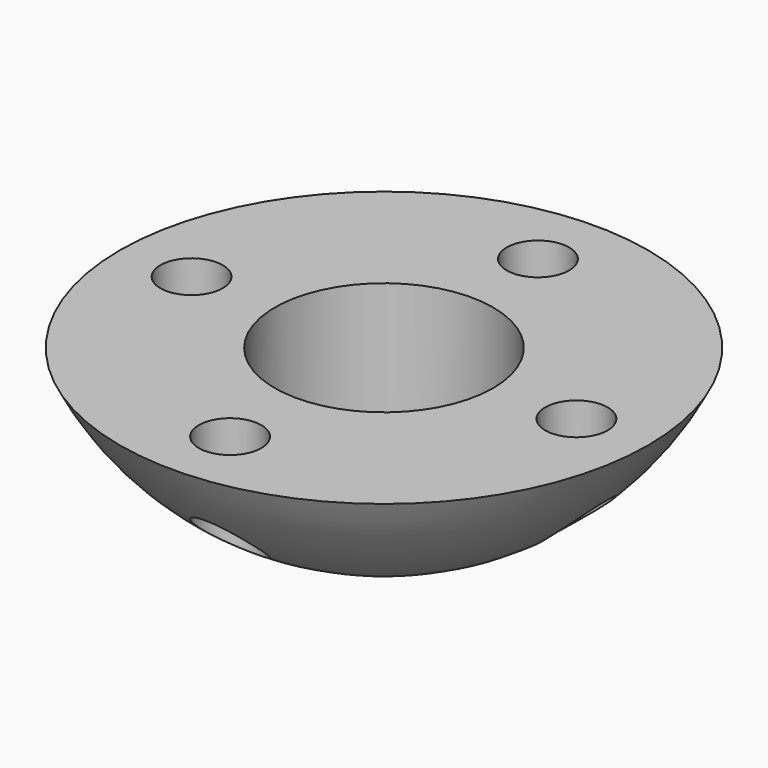
from build123d import *

# Parameters (mm, degrees)
F3_DEPTH = 18
F4_R     = 1.905
F4_R_2   = 6.6675
F5_DEPTH = 10.001


# Not quite as in the source:
# - a feature names something its author has since deleted; it is built from what else it names


with BuildPart() as f1:
    # F0 (on Front) → F1 (revolve)
    with BuildSketch(Plane.XZ):
        with BuildLine():
            Line((0, 18), (0, -18))
            ThreePointArc((0, -18), (18, 0), (0, 18))
        make_face()
    revolve(axis=Axis((0, 0, 0), (0, 0, -1)))

    # F2 (on Right) → F3 (cut, symmetric)
    with BuildSketch(Plane.YZ):
        with BuildLine():
            Line((-16.1245154966, -8), (16.1245154966, -8))
            ThreePointArc((16.1245154966, -8), (0, 18), (-16.1245154966, -8))
        make_face()
    extrude(amount=F3_DEPTH, both=True, mode=Mode.SUBTRACT)

    # F4 (on face) → F5 (cut, through all)
    with BuildSketch(Plane.XY.offset(-8)):
        with Locations((0, -11.7475)):
            Circle(F4_R)
        with Locations((11.7475, 0)):
            Circle(F4_R)
        with Locations((0, 11.7475)):
            Circle(F4_R)
        with Locations((-11.7475, 0)):
            Circle(F4_R)
        Circle(F4_R_2)
    extrude(amount=-F5_DEPTH, mode=Mode.SUBTRACT)


solid = f1.part
